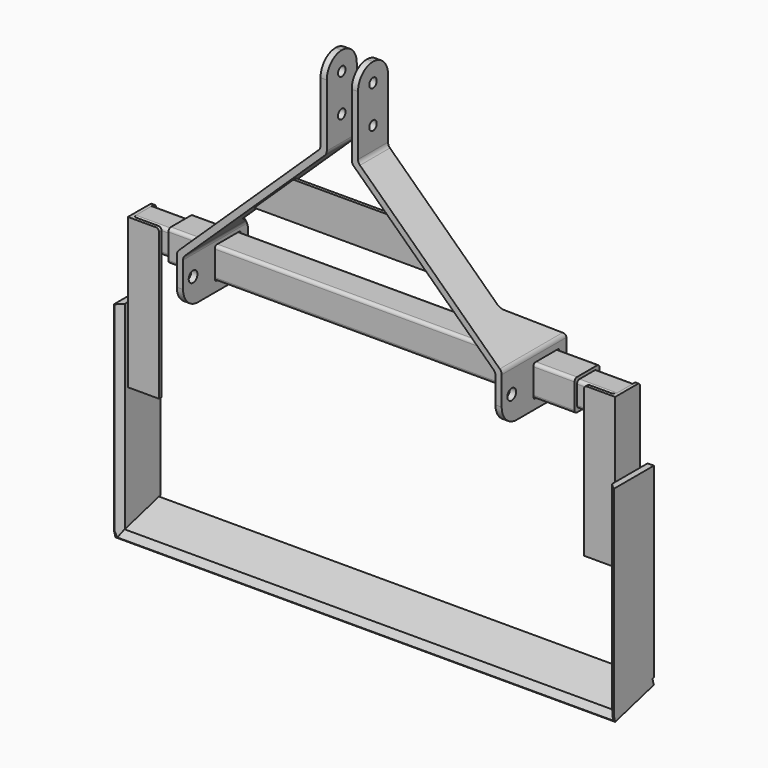
from build123d import *

# Parameters (mm, degrees)
F1_W         = 12.7
F1_H         = 76.2
F4_DEPTH     = 88.9
F6_DEPTH     = 284.1060751771
F7_R         = 12.7
F8_R         = 38.09999
F9_R         = 9.525
F10_DEPTH    = 12.7
F11_R        = 11.1125
F12_DEPTH    = 12.7
F13_R        = 19.05
F14_W        = 64.77
F14_H        = 64.77
F15_DEPTH    = 12.7
F16_R        = 3.175
F18_W        = 63.5
F18_H        = 63.5
F18_W_2      = 50.8
F18_H_2      = 50.8
F19_DEPTH    = 412.75
F20_R        = 6.35
F22_DEPTH    = 6.35
F23_W        = 38.1
F23_H        = 38.1
F24_DEPTH    = 488.95
F25_T1_DEPTH = 69.85
F27_DEPTH    = 304.8
F28_R        = 6.35
F31_DEPTH    = 12.7
F33_W        = 1016
F33_H        = 101.6
F34_DEPTH    = 12.7
F35_SIZE     = 11.43
F36_SIZE     = 11.43


# Not quite as in the source:
# - a fillet or chamfer that OpenCascade refuses, or shapes differently, is made with other operations: its cross-section is extruded or revolved along the edge and cut away or added
# - a fillet or chamfer is up to 0.001 mm smaller than in the source, because OpenCascade refuses the exact size


with BuildPart() as f2:
    # F2: sweep along a path in F0
    with BuildLine(Plane.XZ) as f2_path:
        Line((-330.2, 0), (-330.2, 101.6))
        Line((-330.2, 101.6), (-38.1, 381))
        Line((-38.1, 381), (-38.1, 546.1))
    # F1 (on Top) → F2 (sweep)
    with BuildSketch(Plane.XY):
        with Locations((-323.85, 0)):
            Rectangle(F1_W, F1_H)
    sweep(path=f2_path.line, transition=Transition.RIGHT)

    # F3 (on face) → F4 (join)
    with BuildSketch(Plane(origin=(0, 38.1, 0), x_dir=(-1, 0, 0), z_dir=(0, 1, 0))):
        Polygon((330.2, 0), (330.2, 101.6), (265.9571388996, 163.0496932265), (257.1786112958, 153.8721416407), (317.5, 96.1734220106), (317.5, 0), align=None)
    extrude(amount=F4_DEPTH)

    # F5 (on face) → F6 (cut, through all)
    with BuildSketch(Plane(origin=(-208.5156959526, 0, 217.9936821323), x_dir=(0.7226418571, 0, 0.691222646), z_dir=(-0.691222646, 0, 0.7226418571))):
        Polygon((-79.4881203999, 38.1), (-79.4881203999, 127), (-168.3881203999, 127), align=None)
    extrude(amount=-F6_DEPTH, mode=Mode.SUBTRACT)

    # F7
    f7_edges = [f2.edges().sort_by_distance(p)[0] for p in [
        (-330.2, 44.45, 101.6),
        (-317.5, 41.736711, 96.173422),
        (-38.1, 0, 381),
        (-25.4, 0, 375.573422),
    ]]
    fillet(f7_edges, radius=F7_R)

    # F8 (radius 38.1 in the source; OpenCascade refuses exactly that, so slightly less here)
    f8_edges = [f2.edges().sort_by_distance(p)[0] for p in [
        (-31.75, -38.1, 546.1),
        (-31.75, 38.1, 546.1),
        (-323.85, -38.1, 0),
    ]]
    fillet(f8_edges, radius=F8_R)

    # F9 (on face) → F10 (cut, through all)
    with BuildSketch(Plane(origin=(-38.1, 0, 0), x_dir=(0, -1, 0), z_dir=(-1, 0, 0))):
        with Locations((0, 508)):
            Circle(F9_R)
        with Locations((0, 431.8)):
            Circle(F9_R)
    extrude(amount=-F10_DEPTH, mode=Mode.SUBTRACT)

    # F11 (on face) → F12 (cut, through all)
    with BuildSketch(Plane(origin=(-330.2, 0, 0), x_dir=(0, -1, 0), z_dir=(-1, 0, 0))):
        with Locations((12.7, 50.8)):
            Circle(F11_R)
    extrude(amount=-F12_DEPTH, mode=Mode.SUBTRACT)

    # F13
    f13_edges = [f2.edges().sort_by_distance(p)[0] for p in [
        (-323.85, 127, 0),
        (-323.429135, 127, 94.521368),
        (-261.567875, 38.1, 158.460917),
    ]]
    fillet(f13_edges, radius=F13_R)

    # F14 (on face) → F15 (cut, through all)
    with BuildSketch(Plane(origin=(-330.2, 0, 0), x_dir=(0, -1, 0), z_dir=(-1, 0, 0))):
        with Locations((-75.565, 51.435)):
            Rectangle(F14_W, F14_H)
    extrude(amount=-F15_DEPTH, mode=Mode.SUBTRACT)

    # F16
    f16_edges = [f2.edges().sort_by_distance(p)[0] for p in [
        (-323.85, 107.95, 83.82),
        (-323.85, 43.18, 83.82),
        (-323.85, 43.18, 19.05),
        (-323.85, 107.95, 19.05),
    ]]
    fillet(f16_edges, radius=F16_R)


with BuildPart() as f17_1:
    # F17: instance of F2
    add(f2.part.mirror(Plane.YZ))


with BuildPart() as f19:
    # F18 (on Right) → F19 (new body, symmetric)
    with BuildSketch(Plane.YZ):
        with Locations((75.565, 51.435)):
            Rectangle(F18_W, F18_H)
        with Locations((75.565, 51.435)):
            Rectangle(F18_W_2, F18_H_2, mode=Mode.SUBTRACT)
    extrude(amount=F19_DEPTH, both=True)

    # F20
    f20_edges = [f19.edges().sort_by_distance(p)[0] for p in [
        (0, 100.965, 76.835),
        (0, 50.165, 76.835),
        (0, 50.165, 26.035),
        (0, 100.965, 26.035),
        (0, 43.815, 83.185),
        (0, 43.815, 19.685),
        (0, 107.315, 19.685),
        (0, 107.315, 83.185),
    ]]
    fillet(f20_edges, radius=F20_R)


with BuildPart() as f22:
    # F21 (on Front) → F22 (new body)
    with BuildSketch(Plane.XZ):
        Polygon((-118.6424411929, 286.385), (-198.3060775565, 210.185), (198.3060775565, 210.185), (118.6424411929, 286.385), align=None)
    extrude(amount=F22_DEPTH)


with BuildPart() as f24:
    # F23 (on Right) → F24 (new body, symmetric)
    with BuildSketch(Plane.YZ):
        with BuildLine():
            ThreePointArc((100.965, 70.485), (99.1051280605, 74.9751280605), (94.615, 76.835))
            Line((94.615, 76.835), (56.515, 76.835))
            ThreePointArc((56.515, 76.835), (52.0248719395, 74.9751280605), (50.165, 70.485))
            Line((50.165, 70.485), (50.165, 32.385))
            ThreePointArc((50.165, 32.385), (52.0248719395, 27.8948719395), (56.515, 26.035))
            Line((56.515, 26.035), (94.615, 26.035))
            ThreePointArc((94.615, 26.035), (99.1051280605, 27.8948719395), (100.965, 32.385))
            Line((100.965, 32.385), (100.965, 70.485))
        make_face()
        with Locations((75.565, 51.435)):
            Rectangle(F23_W, F23_H, mode=Mode.SUBTRACT)
    extrude(amount=F24_DEPTH, both=True)

    # F25: fillet of radius 6.35 on 2 edges, made by hand

    # F25_s2 → F25_t1 (cut)
    with BuildSketch(Plane.XY.offset(16.51)):
        with BuildLine():
            ThreePointArc((-482.6, 50.165), (-487.0901280605, 52.0248719395), (-488.95, 56.515))
            Line((-488.95, 56.515), (-488.95, 50.165))
            Line((-488.95, 50.165), (-482.6, 50.165))
        make_face()
        with BuildLine():
            ThreePointArc((482.6, 50.165), (487.0901280605, 52.0248719395), (488.95, 56.515))
            Line((488.95, 56.515), (488.95, 50.165))
            Line((488.95, 50.165), (482.6, 50.165))
        make_face()
    extrude(amount=F25_T1_DEPTH, mode=Mode.SUBTRACT)


with BuildPart() as f27:
    # F26 (on face) → F27 (new body)
    with BuildSketch(Plane.XY.offset(76.835)):
        with BuildLine():
            Line((-431.8, 43.815), (-431.8, 50.165))
            Line((-431.8, 50.165), (-482.6, 50.165))
            ThreePointArc((-482.6, 50.165), (-487.0901280605, 52.0248719395), (-488.95, 56.515))
            Line((-488.95, 56.515), (-488.95, 107.315))
            Line((-488.95, 107.315), (-495.3, 107.315))
            Line((-495.3, 107.315), (-495.3, 43.815))
            Line((-495.3, 43.815), (-431.8, 43.815))
        make_face()
    extrude(amount=-F27_DEPTH)

    # F28
    f28_edges = [f27.edges().sort_by_distance(p)[0] for p in [
        (-431.8, 46.99, 76.835),
        (-492.125, 107.315, 76.835),
        (-492.125, 107.315, -227.965),
    ]]
    fillet(f28_edges, radius=F28_R)


with BuildPart() as f29_1:
    # F29: instance of F27
    add(f27.part.mirror(Plane.YZ))


with BuildPart() as f31:
    # F30 (on face) → F31 (new body)
    with BuildSketch(Plane.YZ.offset(495.3)):
        Polygon((126.365, -454.741362049), (126.365, -75.565), (24.765, -75.565), (24.765, -481.965), align=None)
    extrude(amount=F31_DEPTH)


with BuildPart() as f27_1:
    add(f27.part)

    # F32: F31 across plane
    add(f31.part.mirror(Plane.YZ))

    add(f31.part)  # F34 merges F31
    # F33 (on face) → F34 (join)
    with BuildSketch(Plane(origin=(0, 122.1501904376, -455.8707168675), x_dir=(1, 0, 0), z_dir=(0, 0.2588190451, -0.9659258263))):
        with Locations((0, 50.0205679848)):
            Rectangle(F33_W, F33_H)
    extrude(amount=F34_DEPTH)

    # F35
    f35_edges = [f27_1.edges().sort_by_distance(p)[0] for p in [
        (-495.3, 24.765, -278.765),
        (495.3, 24.765, -278.765),
    ]]
    chamfer(f35_edges, length=F35_SIZE)

    # F36
    f36_edges = [f27_1.edges().sort_by_distance(p)[0] for p in [
        (501.015, 24.765, -481.965),
        (0, 24.765, -481.965),
        (-501.015, 24.765, -481.965),
    ]]
    chamfer(f36_edges, length=F36_SIZE)


solid = Compound([f2.part, f17_1.part, f19.part, f22.part, f24.part, f29_1.part, f27_1.part])
